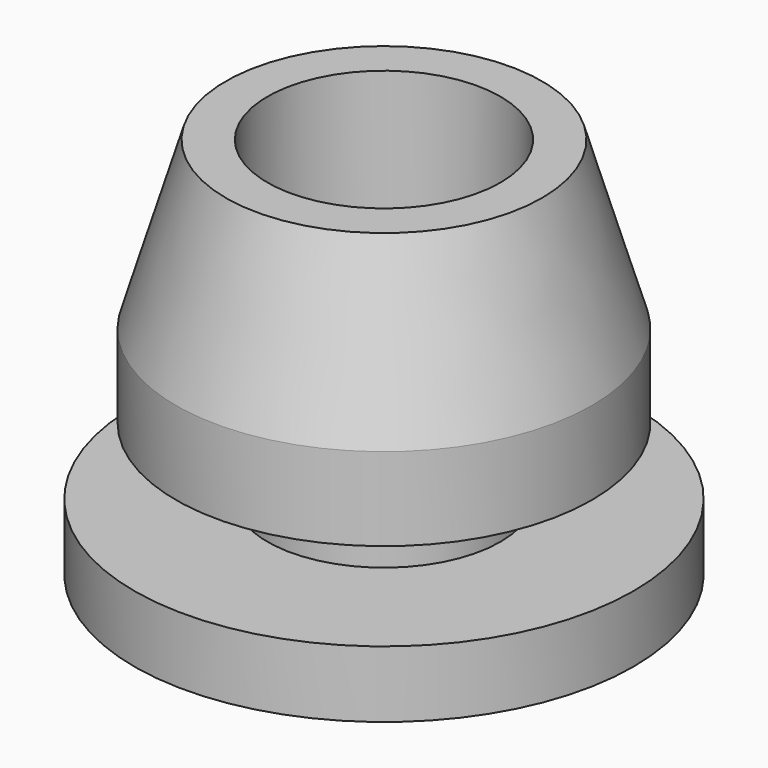
from build123d import *

# Parameters (mm, degrees)
F0_R     = 15
F1_DEPTH = 4
F2_R     = 7
F3_DEPTH = 4
F4_R     = 12.5
F4_R_2   = 7
F5_DEPTH = 15
F6_SIZE2 = 10
F6_SIZE  = 3


# Not quite as in the source:
# - a feature of the source that left no trace in its solid (it failed there, or was rolled back) is left out


with BuildPart() as f1:
    # F0 (on Top) → F1 (new body)
    with BuildSketch(Plane.XY):
        Circle(F0_R)
    extrude(amount=F1_DEPTH)

    # F2 (on face) → F3 (join)
    with BuildSketch(Plane.XY.offset(4)):
        Circle(F2_R)
    extrude(amount=F3_DEPTH)


with BuildPart() as f5:
    # F4 (on face) → F5 (new body)
    with BuildSketch(Plane.XY.offset(8)):
        Circle(F4_R)
        Circle(F4_R_2, mode=Mode.SUBTRACT)
    extrude(amount=F5_DEPTH)

    # F6
    f6_edges = [f5.edges().sort_by_distance(p)[0] for p in [
        (-12.5, 0, 23),
    ]]
    f6_side = f5.faces().sort_by_distance((-12.146447, 0, 23))[0]
    chamfer(f6_edges, length=F6_SIZE, length2=F6_SIZE2, reference=f6_side)


solid = Compound([f1.part, f5.part])
